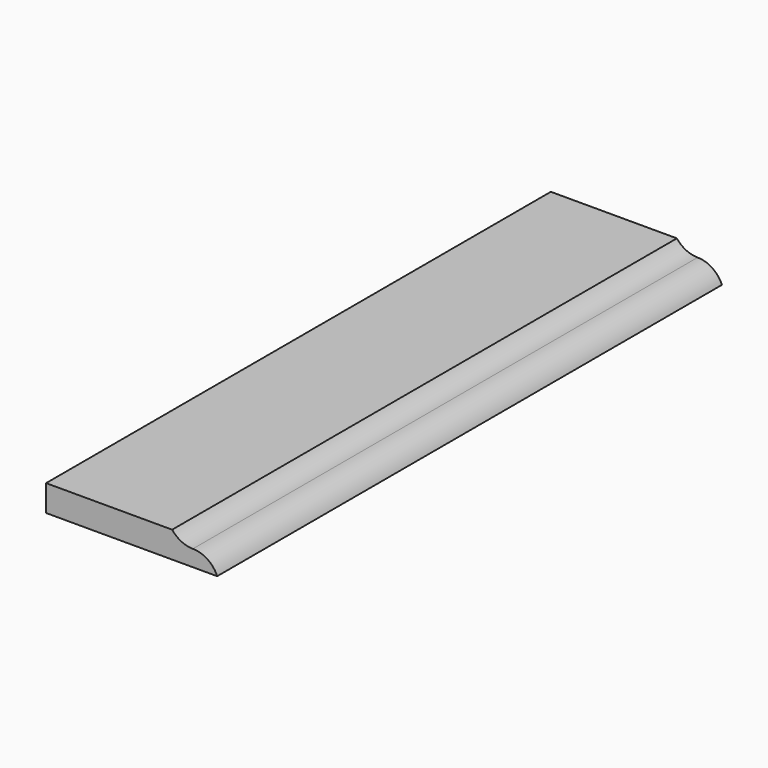
from build123d import *

# Parameters (mm, degrees)
F1_DEPTH = 152.4


# Not quite as in the source:
# - ends of sketch curves that miss each other by under 0.0002 mm in the source are joined


with BuildPart() as f1:
    # F0 (on Front) → F1 (new body)
    with BuildSketch(Plane.XZ):
        with BuildLine():
            ThreePointArc((14.7938744, 0.7382764), (12.0081110559, 1.3810143829), (9.7855278, 3.1792672))
            Line((9.7855278, 3.1792672), (-20.665186, 3.1792672))
            Line((-20.665186, 3.1792672), (-20.665186, -3.1792672))
            Line((-20.665186, -3.1792672), (20.6652114, -3.1792672))
            ThreePointArc((20.6652114, -3.1792672), (18.3230324667, -0.331016316), (14.7938744, 0.7382764))
        make_face()
    extrude(amount=F1_DEPTH)


solid = f1.part
